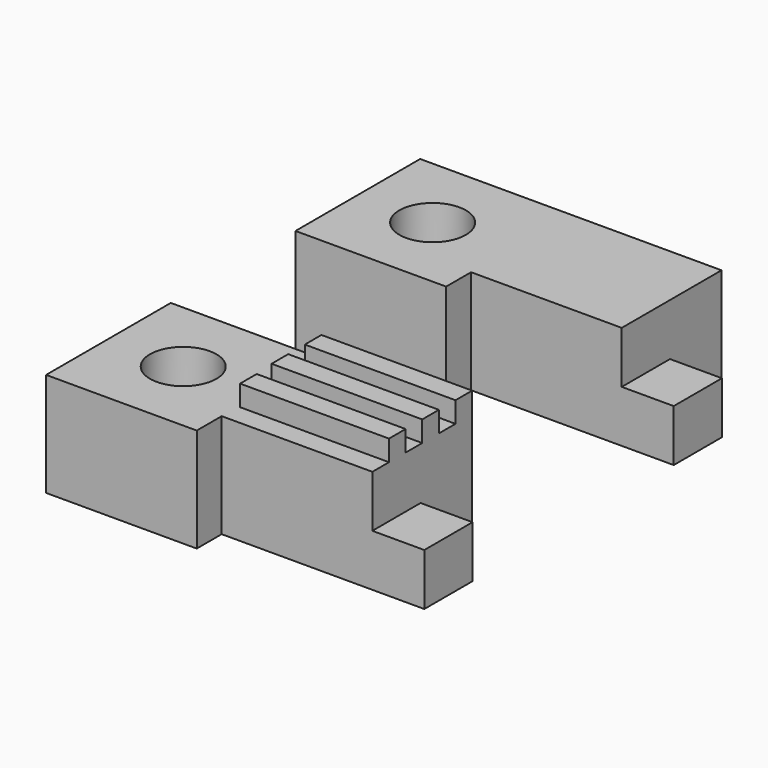
from build123d import *

# Parameters (mm, degrees)
F0_R     = 1.6
F1_DEPTH = 5
F2_W     = 2.9
F2_H     = 2.5
F3_DEPTH = 2.5
F4_R     = 3.1
F4_R_2   = 1.6
F5_DEPTH = 2
F7_W     = 7.25
F7_H     = 1
F7_W_2   = 7.1653089933
F8_DEPTH = 1


with BuildPart() as f1:
    # F0 (on Top) → F1 (new body)
    with BuildSketch(Plane.XY):
        Polygon((0, 7.5), (0, 0), (7.25, 0), (7.25, 1.5), (14.5, 1.5), (14.5, 7.5), align=None)
        with Locations((3.6, 3.75)):
            Circle(F0_R, mode=Mode.SUBTRACT)
    extrude(amount=F1_DEPTH)

    # F2 (on face) → F3 (join)
    with BuildSketch(Plane.YZ.offset(14.5)):
        with Locations((2.95, 1.25)):
            Rectangle(F2_W, F2_H)
    extrude(amount=F3_DEPTH)

    # F4 (on face) → F5 (cut)
    with BuildSketch(Plane(origin=(0, 0, 0), x_dir=(1, 0, 0), z_dir=(0, 0, -1))):
        with Locations((3.6, -3.75)):
            Circle(F4_R)
        with Locations((3.6, -3.75)):
            Circle(F4_R_2, mode=Mode.SUBTRACT)
    extrude(amount=-F5_DEPTH, mode=Mode.SUBTRACT)


with BuildPart() as f6_1:
    # F6: copy of F1
    add(f1.part.moved(Location((0, -15, 0))))

    # F7 (on face) → F8 (join)
    with BuildSketch(Plane.XY.offset(5)):
        with Locations((10.875, -8)):
            Rectangle(F7_W, F7_H)
        with Locations((10.875, -10)):
            Rectangle(F7_W, F7_H)
        with Locations((10.9173455033, -12)):
            Rectangle(F7_W_2, F7_H)
    extrude(amount=F8_DEPTH)


solid = Compound([f1.part, f6_1.part])
